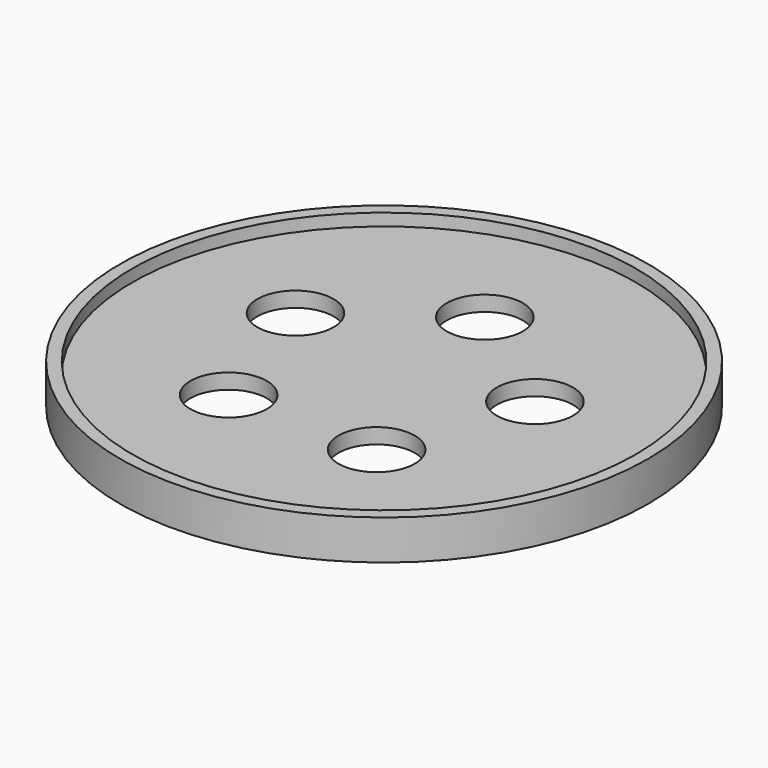
from build123d import *

# Parameters (mm, degrees)
F0_R          = 17.3
F0_R_2        = 16.5
F1_DEPTH      = 1.3
F1_DEPTH_BACK = 1.3
F2_R          = 17.25
F3_DEPTH      = 0.5
F3_DEPTH_BACK = 0.5
F4_R          = 2.5
F5_DEPTH      = 1
F5_DEPTH_BACK = 1


with BuildPart() as f1:
    # F0 (on Top) → F1 (new body, two sides)
    with BuildSketch(Plane.XY) as f1_sk:
        Circle(F0_R)
        Circle(F0_R_2, mode=Mode.SUBTRACT)
    extrude(amount=F1_DEPTH)
    extrude(f1_sk.sketch, amount=-F1_DEPTH_BACK)

    # F2 (on Top) → F3 (join, two sides)
    with BuildSketch(Plane.XY) as f3_sk:
        Circle(F2_R)
    extrude(amount=F3_DEPTH)
    extrude(f3_sk.sketch, amount=-F3_DEPTH_BACK)

    # F4 (on Top) → F5 (cut, two sides)
    with BuildSketch(Plane.XY) as f5_sk:
        with Locations((0, 8.25)):
            Circle(F4_R)
        with Locations((-7.8462162594, 2.5493902036)):
            Circle(F4_R)
        with Locations((-4.8492283314, -6.6743902036)):
            Circle(F4_R)
        with Locations((4.8492283314, -6.6743902036)):
            Circle(F4_R)
        with Locations((7.8462162594, 2.5493902036)):
            Circle(F4_R)
    extrude(amount=-F5_DEPTH, mode=Mode.SUBTRACT)
    extrude(f5_sk.sketch, amount=F5_DEPTH_BACK, mode=Mode.SUBTRACT)


solid = f1.part
